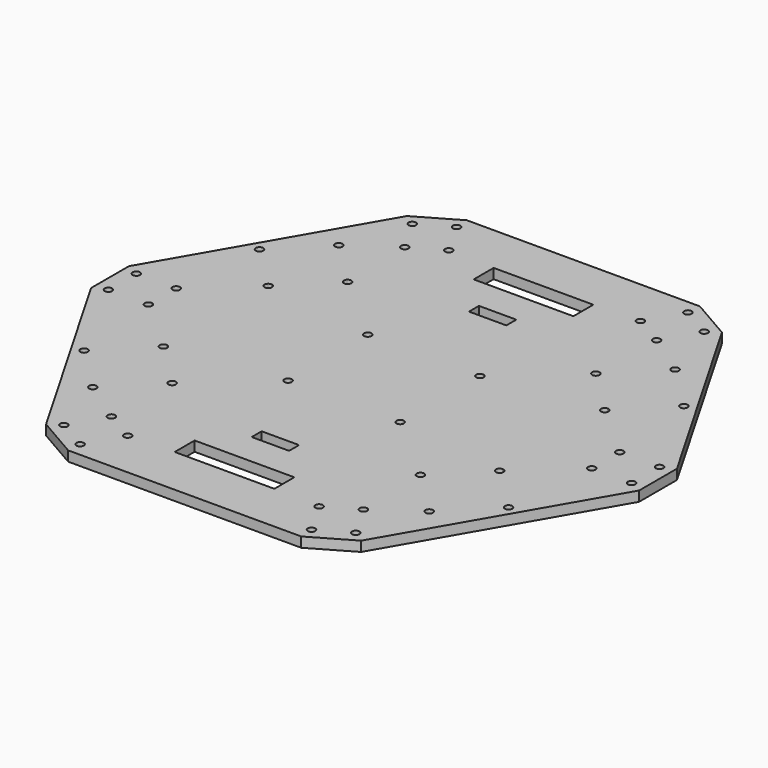
from build123d import *

# Parameters (mm, degrees)
F0_R     = 1.5
F0_W     = 40
F0_H     = 10
F0_W_2   = 15
F0_H_2   = 5
F0_W_3   = 36
F0_H_3   = 40
F0_H_4   = 24
F1_DEPTH = 4


# Not quite as in the source:
# - a feature names something its author has since deleted; it is built from what else it names


with BuildPart() as f1:
    # F0 (on Top) → F1 (new body)
    with BuildSketch(Plane.XY):
        Polygon((-46.7653718044, -100), (46.7653718044, -100), (63.2198544763, -90.5), (109.9852262806, -9.5), (109.9852262806, 9.5), (63.2198544763, 90.5), (46.7653718044, 100), (-46.7653718044, 100), (-54.9926131403, 95.25), (-63.2198544763, 90.5), (-109.9852262806, 9.5), (-109.9852262806, -9.5), (-63.2198544763, -90.5), align=None)
        with Locations((-58.5547909668, -87.4198729811)):
            Circle(F0_R, mode=Mode.SUBTRACT)
        with Locations((-67.5, -61.6776695297)):
            Circle(F0_R, mode=Mode.SUBTRACT)
        with Locations((-46.4304353138, -94.4198729811)):
            Circle(F0_R, mode=Mode.SUBTRACT)
        with Locations((-38.4304353138, -80.5634665205)):
            Circle(F0_R, mode=Mode.SUBTRACT)
        with Locations((-50.5547909668, -73.5634665205)):
            Circle(F0_R, mode=Mode.SUBTRACT)
        with Locations((-85.1776695297, -44)):
            Circle(F0_R, mode=Mode.SUBTRACT)
        with Locations((46.4304353138, -94.4198729811)):
            Circle(F0_R, mode=Mode.SUBTRACT)
        with Locations((38.4304353138, -80.5634665205)):
            Circle(F0_R, mode=Mode.SUBTRACT)
        with Locations((0, -75)):
            Rectangle(F0_W, F0_H, mode=Mode.SUBTRACT)
        with Locations((50.5547909668, -73.5634665205)):
            Circle(F0_R, mode=Mode.SUBTRACT)
        with Locations((58.5547909668, -87.4198729811)):
            Circle(F0_R, mode=Mode.SUBTRACT)
        with Locations((67.5, -61.6776695297)):
            Circle(F0_R, mode=Mode.SUBTRACT)
        with Locations((85.1776695297, -44)):
            Circle(F0_R, mode=Mode.SUBTRACT)
        with Locations((88.9852262806, -7)):
            Circle(F0_R, mode=Mode.SUBTRACT)
        with Locations((104.9852262806, -7)):
            Circle(F0_R, mode=Mode.SUBTRACT)
        with BuildLine():
            Line((-90.4852262806, -7), (-103.4852262806, -7))
            ThreePointArc((-103.4852262806, -7), (-106.0458864524, -8.0606601718), (-104.9852262806, -5.5))
            Line((-104.9852262806, -5.5), (-104.9852262806, 5.5))
            ThreePointArc((-104.9852262806, 5.5), (-106.0458864524, 8.0606601718), (-103.4852262806, 7))
            Line((-103.4852262806, 7), (-90.4852262806, 7))
            ThreePointArc((-90.4852262806, 7), (-88.9852262806, 8.5), (-87.4852262806, 7))
            ThreePointArc((-87.4852262806, 7), (-87.9245661088, 5.9393398282), (-88.9852262806, 5.5))
            Line((-88.9852262806, 5.5), (-88.9852262806, -5.5))
            ThreePointArc((-88.9852262806, -5.5), (-87.9245661088, -5.9393398282), (-87.4852262806, -7))
            ThreePointArc((-87.4852262806, -7), (-88.9852262806, -8.5), (-90.4852262806, -7))
        make_face(mode=Mode.SUBTRACT)
        with BuildLine():
            Line((-48.3223304703, 44), (-18, 44))
            Line((-18, 44), (-18, 52))
            Line((-18, 52), (-7.5, 52))
            Line((-7.5, 52), (-7.5, 57))
            Line((-7.5, 57), (7.5, 57))
            Line((7.5, 57), (7.5, 52))
            Line((7.5, 52), (18, 52))
            Line((18, 52), (18, 44))
            Line((18, 44), (48.3223304703, 44))
            ThreePointArc((48.3223304703, 44), (49.8223304703, 45.5), (51.3223304703, 44))
            Line((51.3223304703, 44), (67.5, 44))
            Line((67.5, 44), (67.5, 27.8223304703))
            ThreePointArc((67.5, 27.8223304703), (68.5606601718, 27.3829906421), (69, 26.3223304703))
            ThreePointArc((69, 26.3223304703), (68.5606601718, 25.2616702986), (67.5, 24.8223304703))
            Line((67.5, 24.8223304703), (67.5, -24.8223304703))
            ThreePointArc((67.5, -24.8223304703), (68.5606601718, -25.2616702986), (69, -26.3223304703))
            ThreePointArc((69, -26.3223304703), (68.5606601718, -27.3829906421), (67.5, -27.8223304703))
            Line((67.5, -27.8223304703), (67.5, -44))
            Line((67.5, -44), (51.3223304703, -44))
            ThreePointArc((51.3223304703, -44), (49.8223304703, -45.5), (48.3223304703, -44))
            Line((48.3223304703, -44), (18, -44))
            Line((18, -44), (18, -52))
            Line((18, -52), (7.5, -52))
            Line((7.5, -52), (7.5, -57))
            Line((7.5, -57), (-7.5, -57))
            Line((-7.5, -57), (-7.5, -52))
            Line((-7.5, -52), (-18, -52))
            Line((-18, -52), (-18, -44))
            Line((-18, -44), (-48.3223304703, -44))
            ThreePointArc((-48.3223304703, -44), (-49.8223304703, -45.5), (-51.3223304703, -44))
            Line((-51.3223304703, -44), (-67.5, -44))
            Line((-67.5, -44), (-67.5, -27.8223304703))
            ThreePointArc((-67.5, -27.8223304703), (-69, -26.3223304703), (-67.5, -24.8223304703))
            Line((-67.5, -24.8223304703), (-67.5, 24.8223304703))
            ThreePointArc((-67.5, 24.8223304703), (-68.8858192988, 25.7483053218), (-68.5606601718, 27.3829906421))
            Line((-68.5606601718, 27.3829906421), (-84.1170093579, 42.9393398282))
            ThreePointArc((-84.1170093579, 42.9393398282), (-86.6776695297, 44), (-84.1170093579, 45.0606601718))
            Line((-84.1170093579, 45.0606601718), (-68.5606601718, 60.6170093579))
            ThreePointArc((-68.5606601718, 60.6170093579), (-68.0740251485, 63.0634888284), (-66, 61.6776695297))
            ThreePointArc((-66, 61.6776695297), (-66.1141807012, 61.1036443811), (-66.4393398282, 60.6170093579))
            Line((-66.4393398282, 60.6170093579), (-50.8829906421, 45.0606601718))
            ThreePointArc((-50.8829906421, 45.0606601718), (-49.2483053218, 45.3858192988), (-48.3223304703, 44))
        make_face(mode=Mode.SUBTRACT)
        with Locations((-58.5547909668, 87.4198729811)):
            Circle(F0_R, mode=Mode.SUBTRACT)
        with Locations((-50.5547909668, 73.5634665205)):
            Circle(F0_R, mode=Mode.SUBTRACT)
        with Locations((-38.4304353138, 80.5634665205)):
            Circle(F0_R, mode=Mode.SUBTRACT)
        with Locations((-46.4304353138, 94.4198729811)):
            Circle(F0_R, mode=Mode.SUBTRACT)
        with Locations((88.9852262806, 7)):
            Circle(F0_R, mode=Mode.SUBTRACT)
        with Locations((104.9852262806, 7)):
            Circle(F0_R, mode=Mode.SUBTRACT)
        with Locations((85.1776695297, 44)):
            Circle(F0_R, mode=Mode.SUBTRACT)
        with Locations((50.5547909668, 73.5634665205)):
            Circle(F0_R, mode=Mode.SUBTRACT)
        with Locations((0, 75)):
            Rectangle(F0_W, F0_H, mode=Mode.SUBTRACT)
        with Locations((38.4304353138, 80.5634665205)):
            Circle(F0_R, mode=Mode.SUBTRACT)
        with Locations((46.4304353138, 94.4198729811)):
            Circle(F0_R, mode=Mode.SUBTRACT)
        with Locations((67.5, 61.6776695297)):
            Circle(F0_R, mode=Mode.SUBTRACT)
        with Locations((58.5547909668, 87.4198729811)):
            Circle(F0_R, mode=Mode.SUBTRACT)
        with BuildLine():
            Line((21, 20), (18, 20))
            Line((18, 20), (18, -20))
            Line((18, -20), (21, -20))
            ThreePointArc((21, -20), (21.4393398282, -18.9393398282), (22.5, -18.5))
            Line((22.5, -18.5), (22.5, 18.5))
            ThreePointArc((22.5, 18.5), (21.4393398282, 18.9393398282), (21, 20))
        make_face()
        Polygon((-18, 52), (-18, 44), (18, 44), (18, 52), (7.5, 52), (7.5, 47), (-7.5, 47), (-7.5, 52), align=None)
        with Locations((0, 49.5)):
            Rectangle(F0_W_2, F0_H_2)
        with BuildLine():
            Line((-18, 20), (-21, 20))
            ThreePointArc((-21, 20), (-21.4393398282, 18.9393398282), (-22.5, 18.5))
            Line((-22.5, 18.5), (-22.5, -18.5))
            ThreePointArc((-22.5, -18.5), (-21.4393398282, -18.9393398282), (-21, -20))
            Line((-21, -20), (-18, -20))
            Line((-18, -20), (-18, 20))
        make_face()
        Polygon((18, -44), (-18, -44), (-18, -52), (-7.5, -52), (-7.5, -47), (7.5, -47), (7.5, -52), (18, -52), align=None)
        Rectangle(F0_W_3, F0_H_3)
        with Locations((0, -49.5)):
            Rectangle(F0_W_2, F0_H_2)
        with BuildLine():
            ThreePointArc((-22.5, 18.5), (-23.5606601718, 21.0606601718), (-21, 20))
            Line((-21, 20), (-18, 20))
            Line((-18, 20), (-18, 44))
            Line((-18, 44), (-48.3223304703, 44))
            ThreePointArc((-48.3223304703, 44), (-49.2483053218, 42.6141807012), (-50.8829906421, 42.9393398282))
            Line((-50.8829906421, 42.9393398282), (-66.4393398282, 27.3829906421))
            ThreePointArc((-66.4393398282, 27.3829906421), (-66.1141807012, 26.8963556189), (-66, 26.3223304703))
            ThreePointArc((-66, 26.3223304703), (-66.4393398282, 25.2616702986), (-67.5, 24.8223304703))
            Line((-67.5, 24.8223304703), (-67.5, -24.8223304703))
            ThreePointArc((-67.5, -24.8223304703), (-66.4393398282, -25.2616702986), (-66, -26.3223304703))
            ThreePointArc((-66, -26.3223304703), (-66.4393398282, -27.3829906421), (-67.5, -27.8223304703))
            Line((-67.5, -27.8223304703), (-67.5, -44))
            Line((-67.5, -44), (-51.3223304703, -44))
            ThreePointArc((-51.3223304703, -44), (-49.8223304703, -42.5), (-48.3223304703, -44))
            Line((-48.3223304703, -44), (-18, -44))
            Line((-18, -44), (-18, -20))
            Line((-18, -20), (-21, -20))
            ThreePointArc((-21, -20), (-23.5606601718, -21.0606601718), (-22.5, -18.5))
            Line((-22.5, -18.5), (-22.5, 18.5))
        make_face()
        with BuildLine():
            ThreePointArc((-51.3223304703, 44), (-51.2081497691, 44.5740251485), (-50.8829906421, 45.0606601718))
            Line((-50.8829906421, 45.0606601718), (-66.4393398282, 60.6170093579))
            ThreePointArc((-66.4393398282, 60.6170093579), (-67.5, 60.1776695297), (-68.5606601718, 60.6170093579))
            Line((-68.5606601718, 60.6170093579), (-84.1170093579, 45.0606601718))
            ThreePointArc((-84.1170093579, 45.0606601718), (-83.7918502309, 44.5740251485), (-83.6776695297, 44))
            ThreePointArc((-83.6776695297, 44), (-83.7918502309, 43.4259748515), (-84.1170093579, 42.9393398282))
            Line((-84.1170093579, 42.9393398282), (-68.5606601718, 27.3829906421))
            ThreePointArc((-68.5606601718, 27.3829906421), (-68.0740251485, 27.7081497691), (-67.5, 27.8223304703))
            Line((-67.5, 27.8223304703), (-67.5, 44))
            Line((-67.5, 44), (-51.3223304703, 44))
        make_face()
        with BuildLine():
            Line((-66.4393398282, 27.3829906421), (-50.8829906421, 42.9393398282))
            ThreePointArc((-50.8829906421, 42.9393398282), (-51.2081497691, 43.4259748515), (-51.3223304703, 44))
            Line((-51.3223304703, 44), (-67.5, 44))
            Line((-67.5, 44), (-67.5, 27.8223304703))
            ThreePointArc((-67.5, 27.8223304703), (-66.9259748515, 27.7081497691), (-66.4393398282, 27.3829906421))
        make_face()
        with BuildLine():
            Line((18, 44), (18, 20))
            Line((18, 20), (21, 20))
            ThreePointArc((21, 20), (22.5, 21.5), (24, 20))
            ThreePointArc((24, 20), (23.5606601718, 18.9393398282), (22.5, 18.5))
            Line((22.5, 18.5), (22.5, -18.5))
            ThreePointArc((22.5, -18.5), (23.5606601718, -18.9393398282), (24, -20))
            ThreePointArc((24, -20), (22.5, -21.5), (21, -20))
            Line((21, -20), (18, -20))
            Line((18, -20), (18, -44))
            Line((18, -44), (48.3223304703, -44))
            ThreePointArc((48.3223304703, -44), (49.8223304703, -42.5), (51.3223304703, -44))
            Line((51.3223304703, -44), (67.5, -44))
            Line((67.5, -44), (67.5, -27.8223304703))
            ThreePointArc((67.5, -27.8223304703), (66, -26.3223304703), (67.5, -24.8223304703))
            Line((67.5, -24.8223304703), (67.5, 24.8223304703))
            ThreePointArc((67.5, 24.8223304703), (66, 26.3223304703), (67.5, 27.8223304703))
            Line((67.5, 27.8223304703), (67.5, 44))
            Line((67.5, 44), (51.3223304703, 44))
            ThreePointArc((51.3223304703, 44), (49.8223304703, 42.5), (48.3223304703, 44))
            Line((48.3223304703, 44), (18, 44))
        make_face()
        with Locations((0, 32)):
            Rectangle(F0_W_3, F0_H_4)
        with Locations((0, -32)):
            Rectangle(F0_W_3, F0_H_4)
        with BuildLine():
            ThreePointArc((-104.9852262806, -5.5), (-103.9245661088, -5.9393398282), (-103.4852262806, -7))
            Line((-103.4852262806, -7), (-90.4852262806, -7))
            ThreePointArc((-90.4852262806, -7), (-90.0458864524, -5.9393398282), (-88.9852262806, -5.5))
            Line((-88.9852262806, -5.5), (-88.9852262806, 5.5))
            ThreePointArc((-88.9852262806, 5.5), (-90.0458864524, 5.9393398282), (-90.4852262806, 7))
            Line((-90.4852262806, 7), (-103.4852262806, 7))
            ThreePointArc((-103.4852262806, 7), (-103.9245661088, 5.9393398282), (-104.9852262806, 5.5))
            Line((-104.9852262806, 5.5), (-104.9852262806, -5.5))
        make_face()
    extrude(amount=F1_DEPTH)


solid = f1.part
